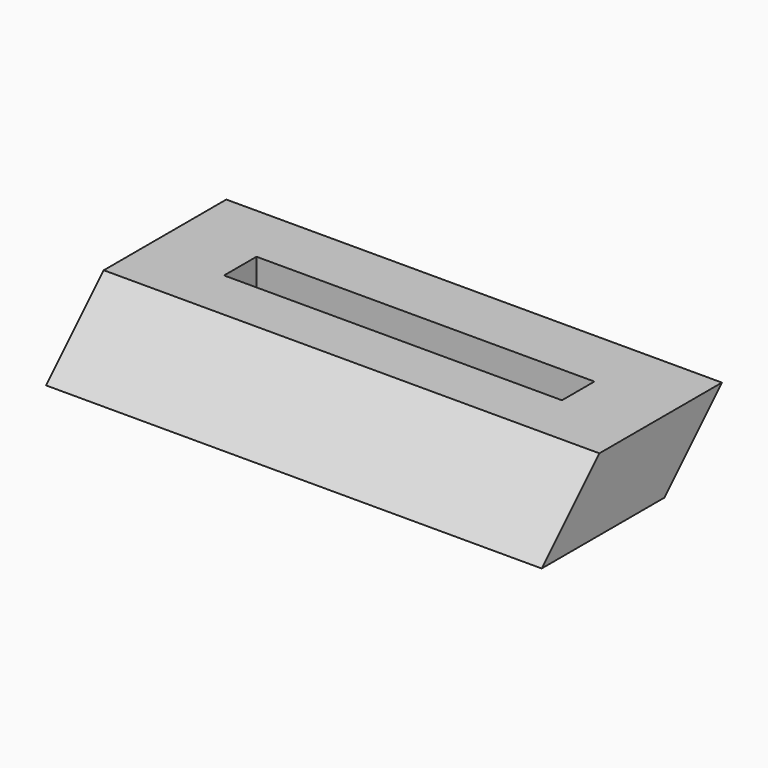
from build123d import *

# Parameters (mm, degrees)
F0_W        = 110
F0_H        = 50
F1_DEPTH    = 16
F2_SIZE     = 15.99999
F3_T1_DEPTH = 192.2938556149


# Not quite as in the source:
# - a fillet or chamfer that OpenCascade refuses, or shapes differently, is made with other operations: its cross-section is extruded or revolved along the edge and cut away or added
# - a fillet or chamfer is up to 0.001 mm smaller than in the source, because OpenCascade refuses the exact size


with BuildPart() as f1:
    # F0 (on Top) → F1 (new body)
    with BuildSketch(Plane.XY):
        with Locations((55, 25)):
            Rectangle(F0_W, F0_H)
        Polygon((17.5, 36.5), (55, 36.5), (92.5, 36.5), (92.5, 27.5), (17.5, 27.5), align=None, mode=Mode.SUBTRACT)
    extrude(amount=F1_DEPTH)

    # F2 (size 16 in the source; OpenCascade refuses exactly that, so slightly less here)
    f2_edges = [f1.edges().sort_by_distance(p)[0] for p in [
        (55, 0, 16),
    ]]
    chamfer(f2_edges, length=F2_SIZE)

    # F3: chamfer of 16 on 1 edges, made by hand

    # F3_s2 → F3_t1 (cut)
    with BuildSketch(Plane.YZ.offset(-41.1469278075)):
        Polygon((34, 0), (50, 16), (50, 0), align=None)
    extrude(amount=F3_T1_DEPTH, mode=Mode.SUBTRACT)


solid = f1.part
